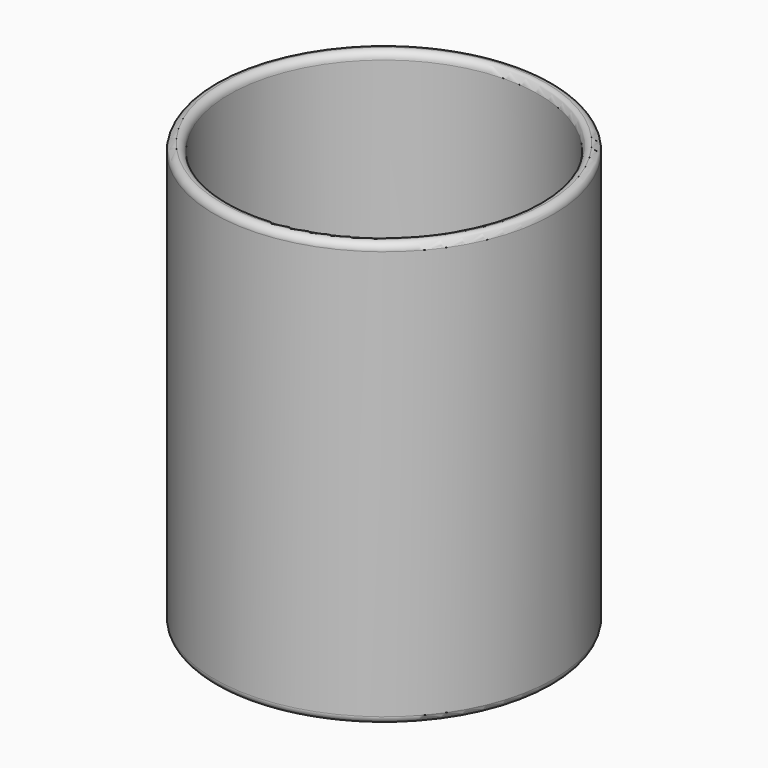
from build123d import *

# Parameters (mm, degrees)
F2_T     = -3.5
F3_R     = 1.74999
F4_R     = 38.25
F5_DEPTH = 3
F6_R     = 1.74999


# Not quite as in the source:
# - a fillet or chamfer that OpenCascade refuses, or shapes differently, is made with other operations: its cross-section is extruded or revolved along the edge and cut away or added
# - a fillet or chamfer is up to 0.001 mm smaller than in the source, because OpenCascade refuses the exact size


with BuildPart() as f1:
    # F0 (on Front) → F1 (revolve)
    with BuildSketch(Plane.XZ):
        with BuildLine():
            Line((0, 100), (0, 0))
            Line((0, 0), (40, 0))
            Line((40, 0), (40, 9.3798986314))
            add(Edge.make_bspline(
                [(40, 9.3798986314), (36.3615811377, 9.5180089921), (32.7559413641, 9.8779920191), (29.1503015906, 10.237975046)],
                knots=[0.9214250826, 0.9214250826, 0.9214250826, 0.9214250826, 1, 1, 1, 1], degree=3))
            Line((29.1503015906, 10.237975046), (30.0444061749, 19.1934501913))
            add(Edge.make_bspline(
                [(40, 18.3365735612), (39.0117054739, 18.370443261), (36.643767227, 18.4954262507), (33.3320197728, 18.8677992603), (31.0010337577, 19.1072868184), (30.0444061749, 19.1934501913)],
                knots=[113.3617815831, 113.3617815831, 113.3617815831, 113.3617815831, 116.3275721529, 120.4741421163, 123.3563956747, 123.3563956747, 123.3563956747, 123.3563956747], degree=3))
            Line((40, 18.3365735612), (40, 73.0902536278))
            add(Edge.make_bspline(
                [(31.7338511682, 71.8869126854), (32.4007501321, 71.9844232047), (34.386427689, 72.278853309), (37.1398587874, 72.6929898238), (39.229939508, 72.9860445189), (40, 73.0902536278)],
                knots=[0, 0, 0, 0, 2.0219920564, 6.0221045926, 8.3532693238, 8.3532693238, 8.3532693238, 8.3532693238], degree=3))
            Line((31.7338511682, 71.8869126854), (30.4177049547, 80.7901546359))
            add(Edge.make_bspline(
                [(30.4177049547, 80.7901546359), (33.6321840052, 81.2653438371), (36.8466630556, 81.7405330383), (40, 82.1441317937)],
                knots=[0, 0, 0, 0, 0.0502198484, 0.0502198484, 0.0502198484, 0.0502198484], degree=3))
            Line((40, 82.1441317937), (40, 100))
            Line((40, 100), (0, 100))
        make_face()
        with BuildLine():
            Line((40, 73.0902536278), (40, 82.1441317937))
            add(Edge.make_bspline(
                [(30.4177049547, 80.7901546359), (33.6321840052, 81.2653438371), (36.8466630556, 81.7405330383), (40, 82.1441317937)],
                knots=[0, 0, 0, 0, 0.0502198484, 0.0502198484, 0.0502198484, 0.0502198484], degree=3))
            Line((30.4177049547, 80.7901546359), (31.7338511682, 71.8869126854))
            add(Edge.make_bspline(
                [(31.7338511682, 71.8869126854), (32.4007501321, 71.9844232047), (34.386427689, 72.278853309), (37.1398587874, 72.6929898238), (39.229939508, 72.9860445189), (40, 73.0902536278)],
                knots=[0, 0, 0, 0, 2.0219920564, 6.0221045926, 8.3532693238, 8.3532693238, 8.3532693238, 8.3532693238], degree=3))
        make_face()
        with BuildLine():
            add(Edge.make_bspline(
                [(40, 9.3798986314), (36.3615811377, 9.5180089921), (32.7559413641, 9.8779920191), (29.1503015906, 10.237975046)],
                knots=[0.9214250826, 0.9214250826, 0.9214250826, 0.9214250826, 1, 1, 1, 1], degree=3))
            Line((40, 9.3798986314), (40, 18.3365735612))
            add(Edge.make_bspline(
                [(40, 18.3365735612), (39.0117054739, 18.370443261), (36.643767227, 18.4954262507), (33.3320197728, 18.8677992603), (31.0010337577, 19.1072868184), (30.0444061749, 19.1934501913)],
                knots=[113.3617815831, 113.3617815831, 113.3617815831, 113.3617815831, 116.3275721529, 120.4741421163, 123.3563956747, 123.3563956747, 123.3563956747, 123.3563956747], degree=3))
            Line((30.0444061749, 19.1934501913), (29.1503015906, 10.237975046))
        make_face()
    revolve(axis=Axis((0, 0, 50), (0, 0, 1)))

    # F2
    f2_openings = [f1.faces().sort_by_distance(p)[0] for p in [
        (0, 0, 100),
    ]]
    offset(amount=F2_T, openings=f2_openings)

    # F3 (radius 1.75 in the source; OpenCascade refuses exactly that, so slightly less here)
    f3_edges = [f1.edges().sort_by_distance(p)[0] for p in [
        (-40, 0, 100),
        (-36.5, 0, 100),
    ]]
    fillet(f3_edges, radius=F3_R)

    # F4 (on Top) → F5 (cut)
    with BuildSketch(Plane.XY):
        Circle(F4_R)
    extrude(amount=F5_DEPTH, mode=Mode.SUBTRACT)

    # F6 (radius 1.75 in the source; OpenCascade refuses exactly that, so slightly less here)
    f6_edges = [f1.edges().sort_by_distance(p)[0] for p in [
        (-40, 0, 0),
    ]]
    fillet(f6_edges, radius=F6_R)

    # F7: fillet of radius 5 on 1 edges, made by hand

    # F7_s1 → F7_t2 (revolve)
    with BuildSketch(Plane.XZ):
        with BuildLine():
            ThreePointArc((38.25, 0), (36.4060370926, 2.1833001327), (33.667424305, 3))
            Line((33.667424305, 3), (38.25, 3))
            Line((38.25, 3), (38.25, 0))
        make_face()
    revolve(axis=Axis((0, 0, 3), (0, 0, 1)))


solid = f1.part
